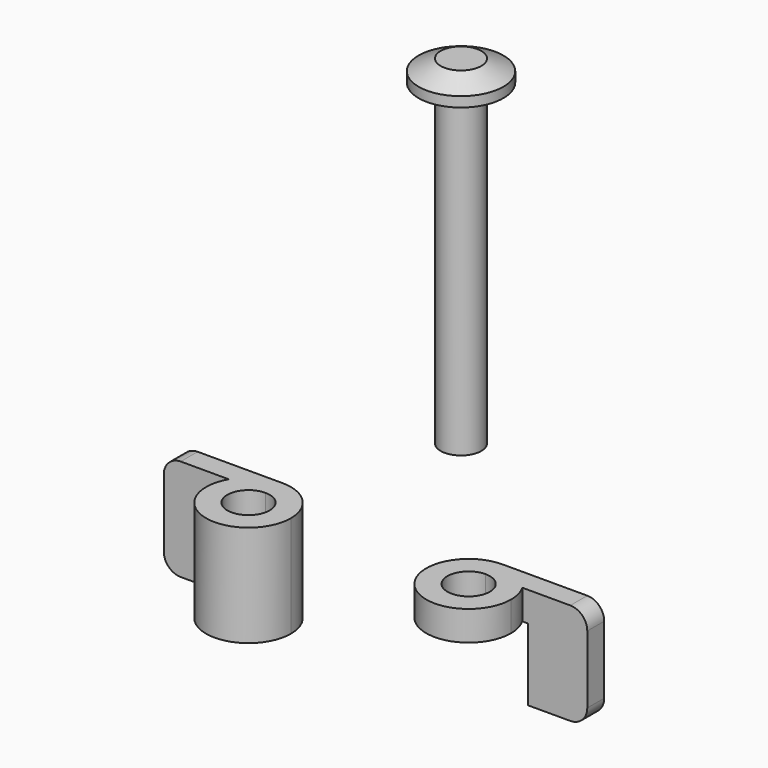
from build123d import *

# Parameters (mm, degrees)
F0_W      = 15.24
F0_H      = 15.24
F1_DEPTH  = 3.175
F3_DEPTH  = 15.24
F5_R      = 2.54
F6_W      = 6.35
F6_H      = 15.24
F7_DEPTH  = 25.4
F8_W      = 15.24
F8_H      = 15.24
F9_DEPTH  = 3.175
F11_DEPTH = 15.24
F12_W     = 12.7
F12_H     = 8.89
F12_W_2   = 6.35
F12_H_2   = 10.795
F13_DEPTH = 25.4
F19_R     = 2.54


# Not quite as in the source:
# - a feature of the source that left no trace in its solid (it failed there, or was rolled back) is left out


with BuildPart() as f1:
    # F0 (on Front) → F1 (new body)
    with BuildSketch(Plane.XZ):
        with Locations((-36.9905814096, -5.1518018644)):
            Rectangle(F0_W, F0_H)
    extrude(amount=F1_DEPTH)

    # F2 (on face) → F3 (join, through all)
    with BuildSketch(Plane.XY.offset(2.4681981356)):
        with BuildLine():
            ThreePointArc((-34.8698427237, -3.175), (-31.014082346, -12.4836289969), (-23.0205814096, -6.35))
            ThreePointArc((-23.0205814096, -6.35), (-24.8804533491, -1.8598719395), (-29.3705814096, 0))
            Line((-29.3705814096, 0), (-29.3705814096, -3.175))
            Line((-29.3705814096, -3.175), (-34.8698427237, -3.175))
        make_face()
        with BuildLine():
            ThreePointArc((-26.1955814096, -6.35), (-31.6156454399, -8.5950640303), (-29.3705814096, -3.175))
            ThreePointArc((-29.3705814096, -3.175), (-27.1255173794, -4.1049359697), (-26.1955814096, -6.35))
        make_face(mode=Mode.SUBTRACT)
        with BuildLine():
            Line((-29.3705814096, -3.175), (-29.3705814096, 0))
            ThreePointArc((-29.3705814096, 0), (-32.5455814096, -0.850738686), (-34.8698427237, -3.175))
            Line((-34.8698427237, -3.175), (-29.3705814096, -3.175))
        make_face()
    extrude(amount=-F3_DEPTH)

    # F5
    f5_edges = [f1.edges().sort_by_distance(p)[0] for p in [
        (-44.610581, -1.5875, 2.468198),
        (-44.610581, -1.5875, -12.771802),
    ]]
    fillet(f5_edges, radius=F5_R)

    # F6 (on face) → F7 (cut)
    with BuildSketch(Plane.XZ):
        with Locations((-32.5455814096, -20.3918018644)):
            Rectangle(F6_W, F6_H)
        with Locations((-26.1955814096, -20.3918018644)):
            Rectangle(F6_W, F6_H)
        Polygon((-35.7205814096, 27.8681981356), (-35.7205814096, 17.7081981356), (-29.3705814096, 17.7081981356), (-29.3705814096, 20.251745157), (-32.0902006372, 27.8681981356), align=None)
        Polygon((-28.4623529462, 17.7081981356), (-23.0205814096, 17.7081981356), (-23.0205814096, 27.8681981356), (-29.3705814096, 27.8681981356), (-29.3705814096, 20.251745157), align=None)
    extrude(amount=F7_DEPTH, mode=Mode.SUBTRACT)


with BuildPart() as f9:
    # F8 (on Front) → F9 (new body)
    with BuildSketch(Plane.XZ):
        with Locations((11.2410542523, -5.1518018644)):
            Rectangle(F8_W, F8_H)
    extrude(amount=F9_DEPTH)

    # F10 (on face) → F11 (join, through all)
    with BuildSketch(Plane.XY.offset(2.4681981356)):
        with BuildLine():
            Line((3.6210542523, -3.175), (3.6210542523, 0))
            ThreePointArc((3.6210542523, 0), (-0.8690738082, -10.8401280605), (9.9710542523, -6.35))
            ThreePointArc((9.9710542523, -6.35), (9.7546832493, -4.7064990636), (9.1203155664, -3.175))
            Line((9.1203155664, -3.175), (3.6210542523, -3.175))
        make_face()
        with BuildLine():
            ThreePointArc((6.7960542523, -6.35), (1.3759902221, -8.5950640303), (3.6210542523, -3.175))
            ThreePointArc((3.6210542523, -3.175), (5.8661182826, -4.1049359697), (6.7960542523, -6.35))
        make_face(mode=Mode.SUBTRACT)
    extrude(amount=-F11_DEPTH)

    # F12 (on face) → F13 (cut)
    with BuildSketch(Plane(origin=(0, 0, 0), x_dir=(-1, 0, 0), z_dir=(0, 1, 0))):
        Polygon((2.7289457477, 18.3431981356), (-9.9710542523, 18.3431981356), (-9.9710542523, 2.4681981356), (-3.6210542523, 2.4681981356), (2.7289457477, 2.4681981356), align=None)
        with Locations((-3.6210542523, 22.7881981356)):
            Rectangle(F12_W, F12_H)
        with Locations((-0.4460542523, -7.3743018644)):
            Rectangle(F12_W_2, F12_H_2)
        with Locations((-6.7960542523, -7.3743018644)):
            Rectangle(F12_W_2, F12_H_2)
    extrude(amount=-F13_DEPTH, mode=Mode.SUBTRACT)

    # F19
    f19_edges = [f9.edges().sort_by_distance(p)[0] for p in [
        (18.861054, -1.5875, 2.468198),
        (18.861054, -1.5875, -12.771802),
    ]]
    fillet(f19_edges, radius=F19_R)


with BuildPart() as f15:
    # F14 (on Front) → F15 (revolve)
    with BuildSketch(Plane.XZ):
        Polygon((-8.9555652812, 64.0162163931), (-5.6535652812, 64.0162163931), (-5.6535652812, 16.3912163931), (-2.6055652812, 16.3912163931), (-2.6055652812, 67.1912163931), (-5.6535652812, 67.1912163931), (-8.9555652812, 65.5202418566), align=None)
    revolve(axis=Axis((-2.6055652812, 0, 41.7912163931), (0, 0, 1)))


solid = Compound([f1.part, f9.part, f15.part])
